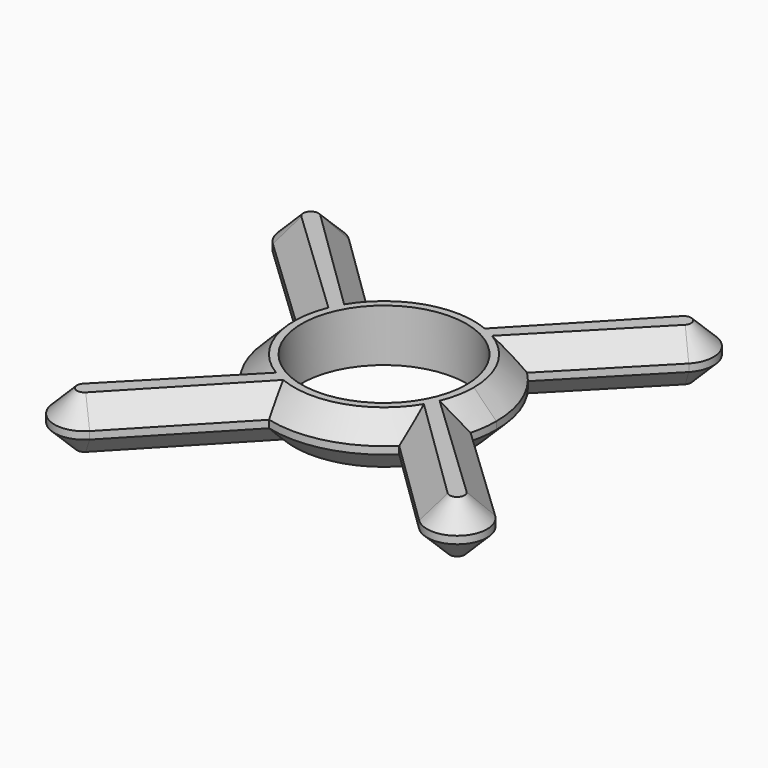
from build123d import *

# Parameters (mm, degrees)
F1_DEPTH = 7
F2_R     = 11
F3_DEPTH = 25
F4_DEPTH = 7
F5_SIZE  = 3
F7_SIZE  = 2.99999


# Not quite as in the source:
# - a fillet or chamfer is up to 0.001 mm smaller than in the source, because OpenCascade refuses the exact size
# - a feature of the source that left no trace in its solid (it failed there, or was rolled back) is left out


with BuildPart() as f1:
    # F0 (on Top) → F1 (new body)
    with BuildSketch(Plane.XY):
        with BuildLine():
            ThreePointArc((-14.5326485793, 3.7151211652), (-13.0157052433, 7.4559651971), (-10.5561338075, 10.6568306282))
            Line((-10.5561338075, 10.6568306282), (-22.7068742866, 22.5203487058))
            ThreePointArc((-22.7068742866, 22.5203487058), (-28.3618988311, 22.3764827918), (-28.2180329171, 16.7214582473))
            Line((-28.2180329171, 16.7214582473), (-14.5326485793, 3.7151211652))
        make_face()
        with BuildLine():
            ThreePointArc((14.5326485793, -3.7151211652), (14.8827035294, -1.872200752), (15, 0))
            ThreePointArc((15, 0), (13.8717781741, 5.7073435404), (10.6568306282, 10.5561338075))
            ThreePointArc((10.6568306282, 10.5561338075), (7.4559651971, 13.0157052433), (3.7151211652, 14.5326485793))
            ThreePointArc((3.7151211652, 14.5326485793), (-3.9313298883, 14.4756569906), (-10.5561338075, 10.6568306282))
            ThreePointArc((-10.5561338075, 10.6568306282), (-13.0157052433, 7.4559651971), (-14.5326485793, 3.7151211652))
            ThreePointArc((-14.5326485793, 3.7151211652), (-14.4756569906, -3.9313298883), (-10.6568306282, -10.5561338075))
            ThreePointArc((-10.6568306282, -10.5561338075), (-7.4559651971, -13.0157052433), (-3.7151211652, -14.5326485793))
            ThreePointArc((-3.7151211652, -14.5326485793), (3.9313298883, -14.4756569906), (10.5561338075, -10.6568306282))
            ThreePointArc((10.5561338075, -10.6568306282), (13.0157052433, -7.4559651971), (14.5326485793, -3.7151211652))
        make_face()
        with BuildLine():
            ThreePointArc((3.7151211652, 14.5326485793), (7.4559651971, 13.0157052433), (10.6568306282, 10.5561338075))
            Line((10.6568306282, 10.5561338075), (22.5203487058, 22.7068742866))
            ThreePointArc((22.5203487058, 22.7068742866), (22.3764827918, 28.3618988311), (16.7214582473, 28.2180329171))
            Line((16.7214582473, 28.2180329171), (3.7151211652, 14.5326485793))
        make_face()
        with BuildLine():
            Line((-16.7214582473, -28.2180329171), (-3.7151211652, -14.5326485793))
            ThreePointArc((-3.7151211652, -14.5326485793), (-7.4559651971, -13.0157052433), (-10.6568306282, -10.5561338075))
            Line((-10.6568306282, -10.5561338075), (-22.5203487058, -22.7068742866))
            ThreePointArc((-22.5203487058, -22.7068742866), (-22.3764827918, -28.3618988311), (-16.7214582473, -28.2180329171))
        make_face()
    extrude(amount=F1_DEPTH)

    # F2 (on face) → F3 (cut)
    with BuildSketch(Plane.XY.offset(7)):
        Circle(F2_R)
    extrude(amount=-F3_DEPTH, mode=Mode.SUBTRACT)

    # F0 (on Top) → F4 (join)
    with BuildSketch(Plane.XY):
        with BuildLine():
            Line((28.2180329171, -16.7214582473), (14.5326485793, -3.7151211652))
            ThreePointArc((14.5326485793, -3.7151211652), (13.0157052433, -7.4559651971), (10.5561338075, -10.6568306282))
            Line((10.5561338075, -10.6568306282), (22.7068742866, -22.5203487058))
            ThreePointArc((22.7068742866, -22.5203487058), (28.3618988311, -22.3764827918), (28.2180329171, -16.7214582473))
        make_face()
    extrude(amount=F4_DEPTH)

    # F5
    f5_edges = [f1.edges().sort_by_distance(p)[0] for p in [
        (16.58859, 16.631504, 7),
        (-16.631504, 16.58859, 7),
        (-16.58859, -16.631504, 7),
        (16.631504, -16.58859, 7),
    ]]
    chamfer(f5_edges, length=F5_SIZE)

    # F7 (size 3 in the source; OpenCascade refuses exactly that, so slightly less here)
    f7_edges = [f1.edges().sort_by_distance(p)[0] for p in [
        (16.631504, -16.58859, 0),
        (3.93133, -14.475657, 0),
        (-10.21829, -21.375341, 0),
        (-16.58859, -16.631504, 0),
        (-14.475657, -3.93133, 0),
        (-21.375341, 10.21829, 0),
        (-16.631504, 16.58859, 0),
        (-28.361899, 22.376483, 0),
        (10.21829, 21.375341, 0),
        (16.58859, 16.631504, 0),
        (22.376483, 28.361899, 0),
        (28.361899, -22.376483, 0),
        (21.375341, -10.21829, 0),
        (-22.376483, -28.361899, 0),
        (-3.93133, 14.475657, 0),
        (14.475657, 3.93133, 0),
        (14.475657, 3.93133, 7),
        (3.93133, -14.475657, 7),
        (-14.475657, -3.93133, 7),
        (-3.93133, 14.475657, 7),
    ]]
    chamfer(f7_edges, length=F7_SIZE)


solid = f1.part
